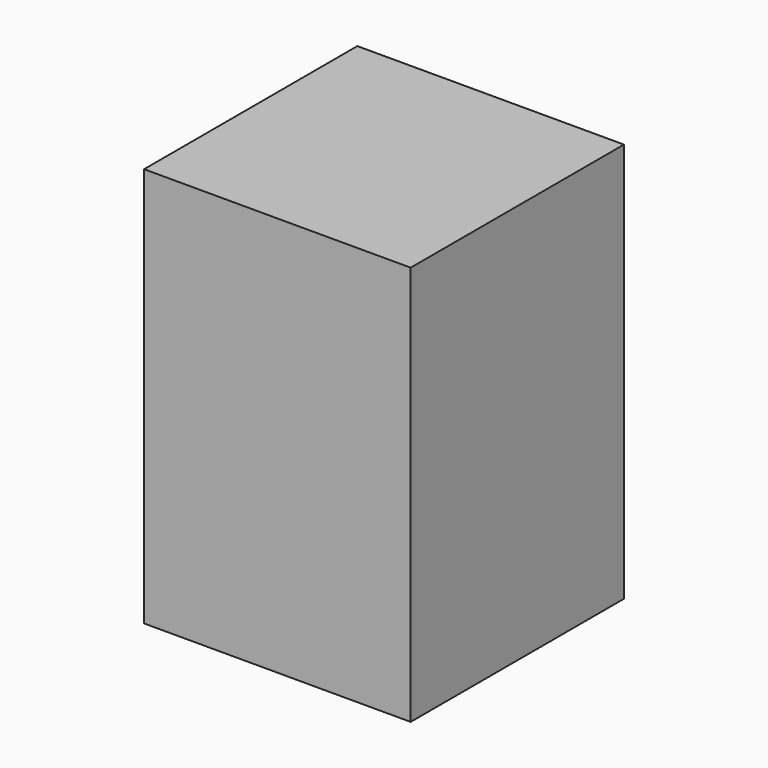
from build123d import *

# Parameters (mm, degrees)
F0_W     = 3.175
F0_H     = 50.8
F0_H_2   = 22.225
F1_DEPTH = 22.225
F2_W     = 3.175
F2_H     = 76.2
F3_DEPTH = 25.4


# Not quite as in the source:
# - a feature names something its author has since deleted; it is built from what else it names


with BuildPart() as f1:
    # F0 (on Front) → F1 (new body, symmetric)
    with BuildSketch(Plane.XZ):
        Polygon((-3.175, 25.4), (0, 25.4), (9.525, 25.4), (12.7, 25.4), (19.4811138548, 25.4), (22.225, 25.4), (25.4, 25.4), (25.4, 28.575), (-25.4, 28.575), (-25.4, 25.4), (-22.225, 25.4), (-15.875, 25.4), (-12.7, 25.4), align=None)
        with Locations((-23.8125, 0)):
            Rectangle(F0_W, F0_H)
        with Locations((-14.2875, 0)):
            Rectangle(F0_W, F0_H)
        with Locations((23.8125, 0)):
            Rectangle(F0_W, F0_H)
        with Locations((11.1125, 0)):
            Rectangle(F0_W, F0_H)
        with Locations((-1.5875, 0)):
            Rectangle(F0_W, F0_H)
        Polygon((25.4, -25.4), (22.225, -25.4), (22.225, -47.625), (25.4, -47.625), (25.4, -39.3581977692), (25.4, -38.6990095903), (25.4, -31.6347628832), align=None)
        with Locations((-23.8125, -36.5125)):
            Rectangle(F0_W, F0_H_2)
    extrude(amount=F1_DEPTH, both=True)

    # F2 (on Right) → F3 (join, symmetric)
    with BuildSketch(Plane.YZ):
        with Locations((-23.8125, -9.525)):
            Rectangle(F2_W, F2_H)
        with Locations((23.8125, -9.525)):
            Rectangle(F2_W, F2_H)
    extrude(amount=F3_DEPTH, both=True)


solid = f1.part
